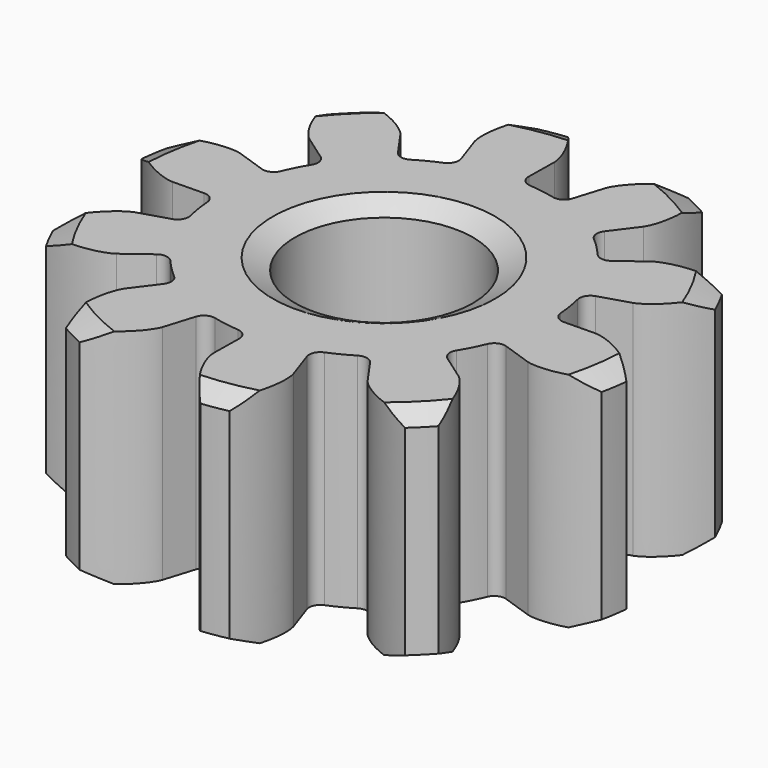
from build123d import *

# Parameters (mm, degrees)
F1_DEPTH   = 5
F2_SIZE2   = 0.25
F2_SIZE    = 0.5
F2_2_SIZE2 = 0.25
F2_2_SIZE  = 0.5
F3_COUNT   = 10
F3_ANGLE   = 324
F0_R       = 2
F4_DEPTH   = 5
F5_SIZE2   = 0.5
F5_SIZE    = 0.25


# Not quite as in the source:
# - ends of sketch curves that miss each other by under 0.0002 mm in the source are joined


with BuildPart() as f1:
    # F0 (on Top) → F1 (new body)
    with BuildSketch(Plane.XY):
        with BuildLine():
            add(Edge.make_bspline(
                [(3.338882, -1.518342), (3.3389573698, -1.5183665545), (3.3393350632, -1.5184901265), (3.3403895153, -1.5188465932), (3.3425230731, -1.5194849147), (3.3459553107, -1.520496218), (3.350790839, -1.5218065621), (3.3570323675, -1.5233965474), (3.3646946351, -1.5252035613), (3.3737853614, -1.5271837464), (3.3843122101, -1.5292884824), (3.3962830167, -1.5314638343), (3.4097018733, -1.5336643681), (3.4245734332, -1.5358369416), (3.4408998865, -1.5379342894), (3.4586828436, -1.5399044522), (3.4779230636, -1.5416956815), (3.4986184496, -1.5432626297), (3.5207671953, -1.5445486213), (3.5443648873, -1.5455089972), (3.5694070717, -1.546091018), (3.5958870308, -1.546243549), (3.6237967464, -1.5459184819), (3.6531269133, -1.5450654103), (3.6838678112, -1.5436339022), (3.7160075436, -1.5415760754), (3.7495332668, -1.5388403595), (3.7844304922, -1.5353802257), (3.8206838474, -1.5311460814), (3.8582761486, -1.5260883878), (3.8971896396, -1.5201610542), (3.9374049759, -1.5133159574), (3.9789010371, -1.5055038404), (4.0216569778, -1.4966819203), (4.0656484991, -1.4867998459), (4.1108525916, -1.4758157388), (4.1572422299, -1.4636806685), (4.2047916803, -1.4503533289), (4.2534724014, -1.4357875673), (4.3032553936, -1.4199392475), (4.3541111405, -1.4027691927), (4.4060073741, -1.3842321098), (4.4589107459, -1.3642859596), (4.5127892339, -1.3428927805), (4.5676079592, -1.3200134763), (4.6233264308, -1.2955990162), (4.6766468783, -1.2711469843), (4.7209052104, -1.2499072408), (4.7495256469, -1.2356683826), (4.7623417749, -1.229235835), (4.765586, -1.227604)],
                knots=[0, 0, 0, 0, 0.0002378066, 0.0011921839, 0.0033390107, 0.0069177312, 0.0119267854, 0.0183673881, 0.0262397616, 0.0355427814, 0.0462777867, 0.0584436965, 0.0720415029, 0.0870700168, 0.1035296592, 0.1214208916, 0.1407425443, 0.1614970119, 0.1836816076, 0.2072972912, 0.232345147, 0.2588246124, 0.2867344584, 0.3160757441, 0.3468478491, 0.3790524177, 0.4126874729, 0.4477541915, 0.4842521421, 0.5221812351, 0.5615414392, 0.6023331673, 0.6445561974, 0.688210082, 0.7332962574, 0.779812719, 0.8277614022, 0.8771406958, 0.9279508106, 0.9801930174, 1.0338670575, 1.0889707984, 1.1455072547, 1.2034742942, 1.2628730725, 1.3237029469, 1.3859634027, 1.4388432844, 1.4709681146, 1.4818626975, 1.4818626975, 1.4818626975, 1.4818626975], degree=3))
            ThreePointArc((4.765586, -1.227604), (4.8186430124, -0.938606987), (4.8574879647, -0.6473589962))
            add(Edge.make_bspline(
                [(3.590454, 0.070025), (3.5905336665, 0.0700252642), (3.5909313347, 0.0700268466), (3.5920447643, 0.0700383773), (3.5942707839, 0.069987284), (3.597847545, 0.069888827), (3.6028510702, 0.0696404673), (3.6092785577, 0.0692231524), (3.6171243677, 0.0685739233), (3.6263824705, 0.0676498339), (3.6370443242, 0.066395575), (3.6491014742, 0.0647688155), (3.6625427249, 0.0627122288), (3.6773579437, 0.0601848592), (3.6935333787, 0.0571335895), (3.7110547757, 0.0535110459), (3.729907078, 0.0492708038), (3.75007367, 0.044365144), (3.771536051, 0.0387439337), (3.7942757962, 0.0323652711), (3.8182720438, 0.0251798215), (3.8435027745, 0.0171421481), (3.8699461258, 0.0082092702), (3.8975771442, -0.0016668768), (3.9263717008, -0.0125263497), (3.9563020069, -0.0244168583), (3.9873422133, -0.0373763621), (4.019461428, -0.0514526397), (4.0526322187, -0.0666817514), (4.0868216405, -0.0831084224), (4.1219987393, -0.1007713054), (4.1581306171, -0.1197086421), (4.1951826011, -0.1399604044), (4.2331191533, -0.1615639683), (4.2719041877, -0.1845561057), (4.3115011957, -0.2089714989), (4.3518704773, -0.234847352), (4.3929741624, -0.2622165304), (4.4347709089, -0.2911132007), (4.4772212226, -0.3215678899), (4.5202808613, -0.3536142649), (4.5639084768, -0.3872811406), (4.6080600046, -0.4225980922), (4.6526906118, -0.4595932054), (4.6977551745, -0.4982937266), (4.7432026143, -0.5387306097), (4.7863574368, -0.5784629745), (4.8218865968, -0.6123392292), (4.8447051262, -0.6347266135), (4.8549065297, -0.6448044675), (4.8574879647, -0.6473589962)],
                knots=[0, 0, 0, 0, 0.0002390021, 0.0011930152, 0.0033402844, 0.0069178551, 0.0119275117, 0.0183679609, 0.0262403463, 0.0355440447, 0.0462789525, 0.0584448321, 0.0720414155, 0.0870698819, 0.1035303553, 0.1214210055, 0.1407430551, 0.1614972714, 0.1836818809, 0.2072985747, 0.2323460252, 0.2588249309, 0.2867347731, 0.3160760206, 0.346849463, 0.3790528499, 0.412688241, 0.4477551405, 0.4842523942, 0.5221817783, 0.5615419904, 0.6023339003, 0.6445570185, 0.6882117178, 0.7332969526, 0.779813824, 0.8277621873, 0.8771407769, 0.9279523943, 0.9801941879, 1.0338671726, 1.0889719149, 1.1455080666, 1.2034751802, 1.2628733663, 1.3237035191, 1.385964238, 1.4388442921, 1.4709685023, 1.4818638064, 1.4818638064, 1.4818638064, 1.4818638064], degree=3))
            Line((3.590454, 0.070025), (2.884249543, 0.0594984834))
            ThreePointArc((2.884249543, 0.0594984834), (2.7120949815, 0.1247227011), (2.6312728588, 0.2901287956))
            ThreePointArc((2.6312728588, 0.2901287956), (2.6397019111, 0.1451732231), (2.642513, 0))
            ThreePointArc((2.642513, 0), (2.5708576636, -0.7295755858), (2.3586300478, -1.4312695802))
            ThreePointArc((2.3586300478, -1.4312695802), (2.4866097566, -1.2989344617), (2.6704938606, -1.2901012423))
            Line((2.6704938606, -1.2901012423), (3.338882, -1.518342))
        make_face()
    extrude(amount=F1_DEPTH)

    # F2
    f2_edges = [f1.edges().sort_by_distance(p)[0] for p in [
        (4.818643, -0.938607, 5),
    ]]
    f2_side = f1.faces().sort_by_distance((3.604202, -0.746258, 5))[0]
    chamfer(f2_edges, length=F2_SIZE, length2=F2_SIZE2, reference=f2_side)

    # F2#2
    f2_2_edges = [f1.edges().sort_by_distance(p)[0] for p in [
        (4.818643, -0.938607, 0),
    ]]
    f2_2_side = f1.faces().sort_by_distance((3.604202, -0.746258, 0))[0]
    chamfer(f2_2_edges, length=F2_2_SIZE, length2=F2_2_SIZE2, reference=f2_2_side)


with BuildPart() as f3_1:
    # F3: instance of F1
    add(f1.part.rotate(Axis((-1.107487, 0, 0), (0, 0, 1)), 1 * F3_ANGLE / (F3_COUNT - 1)))


with BuildPart() as f3_2:
    # F3: instance of F1
    add(f1.part.rotate(Axis((-1.107487, 0, 0), (0, 0, 1)), 2 * F3_ANGLE / (F3_COUNT - 1)))


with BuildPart() as f3_3:
    # F3: instance of F1
    add(f1.part.rotate(Axis((-1.107487, 0, 0), (0, 0, 1)), 3 * F3_ANGLE / (F3_COUNT - 1)))


with BuildPart() as f3_4:
    # F3: instance of F1
    add(f1.part.rotate(Axis((-1.107487, 0, 0), (0, 0, 1)), 4 * F3_ANGLE / (F3_COUNT - 1)))


with BuildPart() as f3_5:
    # F3: instance of F1
    add(f1.part.rotate(Axis((-1.107487, 0, 0), (0, 0, 1)), 5 * F3_ANGLE / (F3_COUNT - 1)))


with BuildPart() as f3_6:
    # F3: instance of F1
    add(f1.part.rotate(Axis((-1.107487, 0, 0), (0, 0, 1)), 6 * F3_ANGLE / (F3_COUNT - 1)))


with BuildPart() as f3_7:
    # F3: instance of F1
    add(f1.part.rotate(Axis((-1.107487, 0, 0), (0, 0, 1)), 7 * F3_ANGLE / (F3_COUNT - 1)))


with BuildPart() as f3_8:
    # F3: instance of F1
    add(f1.part.rotate(Axis((-1.107487, 0, 0), (0, 0, 1)), 8 * F3_ANGLE / (F3_COUNT - 1)))


with BuildPart() as f3_9:
    # F3: instance of F1
    add(f1.part.rotate(Axis((-1.107487, 0, 0), (0, 0, 1)), 9 * F3_ANGLE / (F3_COUNT - 1)))


with BuildPart() as f1_1:
    add(f1.part)

    add(f3_1.part)  # F4 merges F3_1

    add(f3_2.part)  # F4 merges F3_2

    add(f3_3.part)  # F4 merges F3_3

    add(f3_4.part)  # F4 merges F3_4

    add(f3_5.part)  # F4 merges F3_5

    add(f3_6.part)  # F4 merges F3_6

    add(f3_7.part)  # F4 merges F3_7

    add(f3_8.part)  # F4 merges F3_8

    add(f3_9.part)  # F4 merges F3_9
    # F0 (on Top) → F4 (join)
    with BuildSketch(Plane.XY):
        with BuildLine():
            ThreePointArc((2.6312728588, 0.2901287956), (-4.8113182464, 0.5866294385), (2.3586300478, -1.4312695802))
            ThreePointArc((2.3586300478, -1.4312695802), (2.5708576636, -0.7295755858), (2.642513, 0))
            ThreePointArc((2.642513, 0), (2.6397019111, 0.1451732231), (2.6312728588, 0.2901287956))
        make_face()
        with Locations((-1.107487, 0)):
            Circle(F0_R, mode=Mode.SUBTRACT)
    extrude(amount=F4_DEPTH)

    # F5
    f5_edges = [f1_1.edges().sort_by_distance(p)[0] for p in [
        (-3.107487, 0, 5),
        (-3.107487, 0, 0),
    ]]
    f5_side = f1_1.faces().sort_by_distance((-3.107487, 0, 2.5))[0]
    chamfer(f5_edges, length=F5_SIZE, length2=F5_SIZE2, reference=f5_side)


solid = f1_1.part
